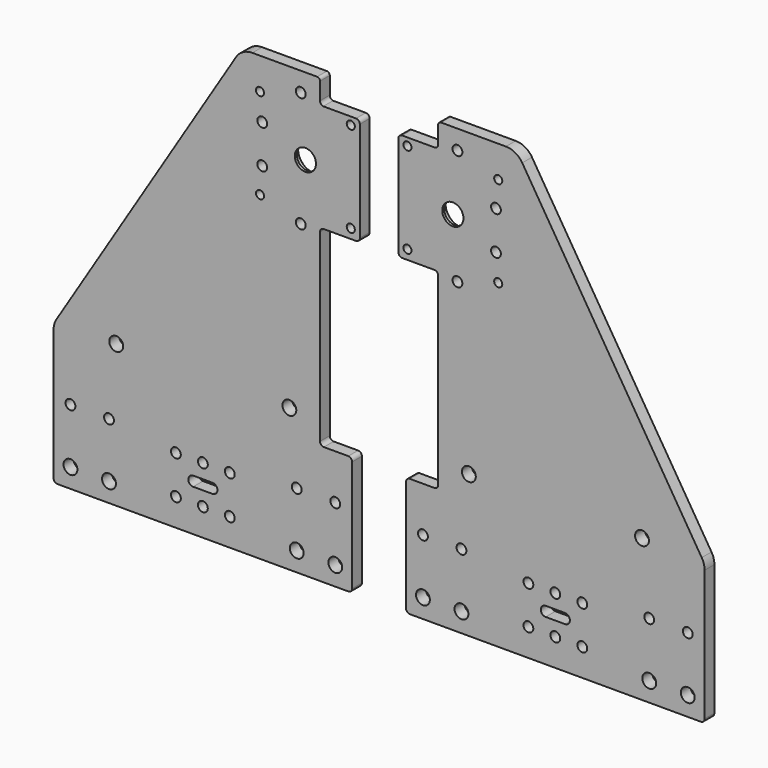
from build123d import *

# Parameters (mm, degrees)
F0_R     = 3.6
F0_R_2   = 2.55
F0_R_3   = 2.1
F0_R_4   = 9.05
F0_R_5   = 8.05
F0_R_6   = 5.5
F1_DEPTH = 6.35
F2_DEPTH = 5
F3_DEPTH = 1
F4_DEPTH = 6.35
F5_DEPTH = 5
F6_DEPTH = 1


# Not quite as in the source:
# - ends of sketch curves that miss each other by under 0.0002 mm in the source are joined


with BuildPart() as f1:
    # F0 (on Front) → F1 (new body)
    with BuildSketch(Plane.XZ):
        with BuildLine():
            Line((-30.674942, -51.12845), (-30.676534, 44.51808))
            ThreePointArc((-30.676534, 44.51808), (-30.2100770853, 45.8287425755), (-29.0016939819, 46.5181108898))
            Line((-29.0016939819, 46.5181108898), (-12.001654, 46.518405))
            ThreePointArc((-12.001654, 46.518405), (-10.5874510427, 47.104215833), (-10.0016890003, 48.518439))
            Line((-10.0016890003, 48.518439), (-10.002565, 100.518439))
            ThreePointArc((-10.002565, 100.518439), (-10.5883751259, 101.9326422503), (-12.002598, 102.5184049997))
            Line((-12.002598, 102.5184049997), (-29.002593, 102.518122))
            ThreePointArc((-29.002593, 102.518122), (-30.2091675508, 103.2084791623), (-30.6743631915, 104.5184440026))
            Line((-30.6743631915, 104.5184440026), (-30.674363, 113.509551))
            ThreePointArc((-30.674363, 113.509551), (-31.1140196595, 114.5705279085), (-32.1752590004, 115.0095507324))
            Line((-32.1752590004, 115.0095507324), (-65.812997, 114.989448))
            ThreePointArc((-65.812997, 114.989448), (-70.670448907, 113.7271299849), (-74.3028867898, 110.2639408695))
            Line((-74.3028867898, 110.2639408695), (-167.496783, -39.847736))
            ThreePointArc((-167.496783, -39.847736), (-168.6175573697, -42.3799245887), (-169.0009169986, -45.122396))
            Line((-169.0009169986, -45.122396), (-168.999774, -113.009551))
            ThreePointArc((-168.999774, -113.009551), (-168.4141982645, -114.4235538289), (-167.00037, -115.0095509112))
            Line((-167.00037, -115.0095509112), (-16.295504, -114.987446))
            ThreePointArc((-16.295504, -114.987446), (-14.6937872777, -114.5249728165), (-13.9989680003, -113.009518))
            Line((-13.9989680003, -113.009518), (-13.999943, -55.128356))
            ThreePointArc((-13.999943, -55.128356), (-14.5857432263, -53.7141626491), (-15.999948, -53.12839))
            Line((-15.999948, -53.12839), (-28.674938, -53.128417))
            ThreePointArc((-28.674938, -53.128417), (-30.0891424808, -52.5426436438), (-30.674942, -51.12845))
        make_face()
        with Locations((-160.24037, -105.009551)):
            Circle(F0_R, mode=Mode.SUBTRACT)
        with Locations((-140.24037, -105.009551)):
            Circle(F0_R, mode=Mode.SUBTRACT)
        with Locations((-105.499813, -100.769551)):
            Circle(F0_R_2, mode=Mode.SUBTRACT)
        with Locations((-91.499813, -100.769551)):
            Circle(F0_R_2, mode=Mode.SUBTRACT)
        with BuildLine():
            Line((-96.49999, -88.219551), (-86.477231, -88.219653))
            ThreePointArc((-86.477231, -88.219653), (-83.927359, -90.769551), (-86.477231, -93.3194489999))
            Line((-86.477231, -93.3194489999), (-96.49999, -93.319551))
            ThreePointArc((-96.49999, -93.319551), (-99.04999, -90.769551), (-96.49999, -88.219551))
        make_face(mode=Mode.SUBTRACT)
        with Locations((-160.24037, -76.509551)):
            Circle(F0_R_2, mode=Mode.SUBTRACT)
        with Locations((-140.24037, -76.509551)):
            Circle(F0_R_2, mode=Mode.SUBTRACT)
        with Locations((-105.500016, -80.769551)):
            Circle(F0_R_2, mode=Mode.SUBTRACT)
        with Locations((-91.500016, -80.769551)):
            Circle(F0_R_2, mode=Mode.SUBTRACT)
        with Locations((-77.499813, -100.769551)):
            Circle(F0_R_2, mode=Mode.SUBTRACT)
        with Locations((-42.759045, -105.009551)):
            Circle(F0_R, mode=Mode.SUBTRACT)
        with Locations((-22.759102, -105.057468)):
            Circle(F0_R, mode=Mode.SUBTRACT)
        with Locations((-77.500016, -80.769551)):
            Circle(F0_R_2, mode=Mode.SUBTRACT)
        with Locations((-42.759525, -76.509551)):
            Circle(F0_R_2, mode=Mode.SUBTRACT)
        with Locations((-22.759582, -76.557468)):
            Circle(F0_R_2, mode=Mode.SUBTRACT)
        with Locations((-136.49037, -41.005075)):
            Circle(F0_R, mode=Mode.SUBTRACT)
        with Locations((-46.595601, -40.99189)):
            Circle(F0_R, mode=Mode.SUBTRACT)
        with Locations((-61.844363, 51.439502)):
            Circle(F0_R_3, mode=Mode.SUBTRACT)
        with Locations((-40.674363, 45.009502)):
            Circle(F0_R_2, mode=Mode.SUBTRACT)
        with Locations((-14.704363, 51.439502)):
            Circle(F0_R_3, mode=Mode.SUBTRACT)
        with Locations((-60.674363, 65.009502)):
            Circle(F0_R_2, mode=Mode.SUBTRACT)
        with Locations((-60.674363, 85.009502)):
            Circle(F0_R_2, mode=Mode.SUBTRACT)
        with Locations((-38.274363, 75.009502)):
            Circle(F0_R_4, mode=Mode.SUBTRACT)
        with Locations((-61.844363, 98.579502)):
            Circle(F0_R_3, mode=Mode.SUBTRACT)
        with Locations((-14.704363, 98.579502)):
            Circle(F0_R_3, mode=Mode.SUBTRACT)
        with Locations((-40.674363, 105.009502)):
            Circle(F0_R_2, mode=Mode.SUBTRACT)
        with Locations((-38.274363, 75.009502)):
            Circle(F0_R_4)
        with Locations((-38.274363, 75.009502)):
            Circle(F0_R_5, mode=Mode.SUBTRACT)
        with Locations((-38.274363, 75.009502)):
            Circle(F0_R_5)
        with Locations((-38.274363, 75.009502)):
            Circle(F0_R_6, mode=Mode.SUBTRACT)
    extrude(amount=F1_DEPTH)

    # F0 (on Front) → F2 (cut)
    with BuildSketch(Plane.XZ):
        with Locations((-38.274363, 75.009502)):
            Circle(F0_R_5)
        with Locations((-38.274363, 75.009502)):
            Circle(F0_R_6, mode=Mode.SUBTRACT)
    extrude(amount=F2_DEPTH, mode=Mode.SUBTRACT)

    # F0 (on Front) → F3 (cut)
    with BuildSketch(Plane.XZ):
        with Locations((-38.274363, 75.009502)):
            Circle(F0_R_4)
        with Locations((-38.274363, 75.009502)):
            Circle(F0_R_5, mode=Mode.SUBTRACT)
    extrude(amount=F3_DEPTH, mode=Mode.SUBTRACT)


with BuildPart() as f4:
    # F0 (on Front) → F4 (new body)
    with BuildSketch(Plane.XZ):
        with BuildLine():
            ThreePointArc((29.0016939819, 46.5181108898), (30.2100770853, 45.8287425755), (30.6765339558, 44.5180800006))
            Line((30.6765339558, 44.5180800006), (30.674942, -51.12845))
            ThreePointArc((30.674942, -51.12845), (30.0891424808, -52.5426436438), (28.674938, -53.128417))
            Line((28.674938, -53.128417), (15.999948, -53.12839))
            ThreePointArc((15.999948, -53.12839), (14.5857432263, -53.7141626491), (13.9999430003, -55.128356))
            Line((13.9999430003, -55.128356), (13.998968, -113.009518))
            ThreePointArc((13.998968, -113.009518), (14.6937872777, -114.5249728165), (16.2955039173, -114.9874454486))
            Line((16.2955039173, -114.9874454486), (167.00037, -115.009551))
            ThreePointArc((167.00037, -115.009551), (168.4141982645, -114.4235538289), (168.999774, -113.009551))
            Line((168.999774, -113.009551), (169.000917, -45.122396))
            ThreePointArc((169.000917, -45.122396), (168.6175573697, -42.3799245887), (167.4967827898, -39.8477361305))
            Line((167.4967827898, -39.8477361305), (74.302887, 110.263941))
            ThreePointArc((74.302887, 110.263941), (70.670448907, 113.7271299849), (65.8129969995, 114.9894472144))
            Line((65.8129969995, 114.9894472144), (32.175259, 115.00955))
            ThreePointArc((32.175259, 115.00955), (31.1140196595, 114.5705279085), (30.674363, 113.509551))
            Line((30.674363, 113.509551), (30.674363, 104.518444))
            ThreePointArc((30.674363, 104.518444), (30.2091675508, 103.2084791623), (29.0025929506, 102.5181222972))
            Line((29.0025929506, 102.5181222972), (12.002598, 102.518405))
            ThreePointArc((12.002598, 102.518405), (10.5883751259, 101.9326422503), (10.0025650003, 100.518439))
            Line((10.0025650003, 100.518439), (10.001689, 48.518439))
            ThreePointArc((10.001689, 48.518439), (10.5874510427, 47.104215833), (12.001654, 46.5184050003))
            Line((12.001654, 46.5184050003), (29.0016939819, 46.5181108898))
        make_face()
        with Locations((22.759102, -105.057468)):
            Circle(F0_R, mode=Mode.SUBTRACT)
        with Locations((42.759045, -105.009551)):
            Circle(F0_R, mode=Mode.SUBTRACT)
        with Locations((77.499813, -100.769551)):
            Circle(F0_R_2, mode=Mode.SUBTRACT)
        with Locations((22.759582, -76.557468)):
            Circle(F0_R_2, mode=Mode.SUBTRACT)
        with Locations((42.759525, -76.509551)):
            Circle(F0_R_2, mode=Mode.SUBTRACT)
        with Locations((77.500016, -80.769551)):
            Circle(F0_R_2, mode=Mode.SUBTRACT)
        with Locations((91.499813, -100.769551)):
            Circle(F0_R_2, mode=Mode.SUBTRACT)
        with Locations((105.499813, -100.769551)):
            Circle(F0_R_2, mode=Mode.SUBTRACT)
        with BuildLine():
            ThreePointArc((86.477231, -93.3194489999), (83.927359, -90.769551), (86.477231, -88.2196530001))
            Line((86.477231, -88.2196530001), (96.49999, -88.219551))
            ThreePointArc((96.49999, -88.219551), (99.04999, -90.769551), (96.49999, -93.319551))
            Line((96.49999, -93.319551), (86.477231, -93.3194489999))
        make_face(mode=Mode.SUBTRACT)
        with Locations((140.24037, -105.009551)):
            Circle(F0_R, mode=Mode.SUBTRACT)
        with Locations((160.24037, -105.009551)):
            Circle(F0_R, mode=Mode.SUBTRACT)
        with Locations((91.500016, -80.769551)):
            Circle(F0_R_2, mode=Mode.SUBTRACT)
        with Locations((105.500016, -80.769551)):
            Circle(F0_R_2, mode=Mode.SUBTRACT)
        with Locations((140.24037, -76.509551)):
            Circle(F0_R_2, mode=Mode.SUBTRACT)
        with Locations((160.24037, -76.509551)):
            Circle(F0_R_2, mode=Mode.SUBTRACT)
        with Locations((46.595601, -40.99189)):
            Circle(F0_R, mode=Mode.SUBTRACT)
        with Locations((136.49037, -41.005075)):
            Circle(F0_R, mode=Mode.SUBTRACT)
        with Locations((14.704363, 51.439502)):
            Circle(F0_R_3, mode=Mode.SUBTRACT)
        with Locations((40.674363, 45.009502)):
            Circle(F0_R_2, mode=Mode.SUBTRACT)
        with Locations((61.844363, 51.439502)):
            Circle(F0_R_3, mode=Mode.SUBTRACT)
        with Locations((38.274363, 75.009502)):
            Circle(F0_R_4, mode=Mode.SUBTRACT)
        with Locations((60.674363, 65.009502)):
            Circle(F0_R_2, mode=Mode.SUBTRACT)
        with Locations((60.674363, 85.009502)):
            Circle(F0_R_2, mode=Mode.SUBTRACT)
        with Locations((14.704363, 98.579502)):
            Circle(F0_R_3, mode=Mode.SUBTRACT)
        with Locations((40.674363, 105.009502)):
            Circle(F0_R_2, mode=Mode.SUBTRACT)
        with Locations((61.844363, 98.579502)):
            Circle(F0_R_3, mode=Mode.SUBTRACT)
        with Locations((38.274363, 75.009502)):
            Circle(F0_R_4)
        with Locations((38.274363, 75.009502)):
            Circle(F0_R_5, mode=Mode.SUBTRACT)
        with Locations((38.274363, 75.009502)):
            Circle(F0_R_5)
        with Locations((38.274363, 75.009502)):
            Circle(F0_R_6, mode=Mode.SUBTRACT)
    extrude(amount=F4_DEPTH)

    # F0 (on Front) → F5 (cut)
    with BuildSketch(Plane.XZ):
        with Locations((38.274363, 75.009502)):
            Circle(F0_R_5)
        with Locations((38.274363, 75.009502)):
            Circle(F0_R_6, mode=Mode.SUBTRACT)
    extrude(amount=F5_DEPTH, mode=Mode.SUBTRACT)

    # F0 (on Front) → F6 (cut)
    with BuildSketch(Plane.XZ):
        with Locations((38.274363, 75.009502)):
            Circle(F0_R_4)
        with Locations((38.274363, 75.009502)):
            Circle(F0_R_5, mode=Mode.SUBTRACT)
    extrude(amount=F6_DEPTH, mode=Mode.SUBTRACT)


solid = Compound([f1.part, f4.part])
